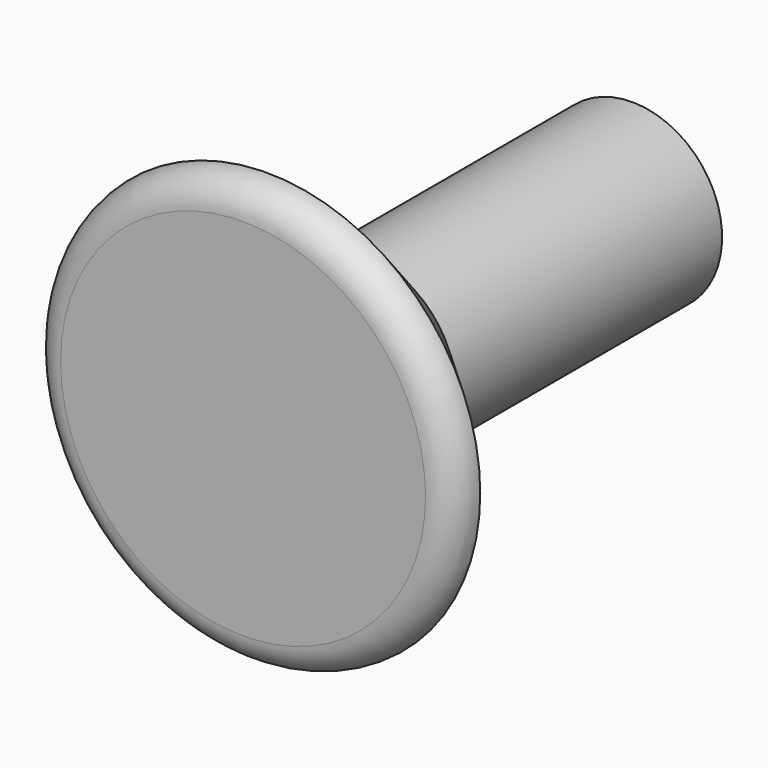
from build123d import *

# Parameters (mm, degrees)
F0_R     = 35
F1_DEPTH = 12.5
F2_R     = 5
F3_SIZE  = 19.99999
F4_R     = 14.7680159512
F5_DEPTH = 55


# Not quite as in the source:
# - a fillet or chamfer is up to 0.001 mm smaller than in the source, because OpenCascade refuses the exact size


with BuildPart() as f1:
    # F0 (on Front) → F1 (new body, symmetric)
    with BuildSketch(Plane.XZ):
        Circle(F0_R)
    extrude(amount=F1_DEPTH, both=True)

    # F2
    f2_edges = [f1.edges().sort_by_distance(p)[0] for p in [
        (-35, -12.5, 0),
    ]]
    fillet(f2_edges, radius=F2_R)

    # F3 (size 20 in the source; OpenCascade refuses exactly that, so slightly less here)
    f3_edges = [f1.edges().sort_by_distance(p)[0] for p in [
        (-35, 12.5, 0),
    ]]
    chamfer(f3_edges, length=F3_SIZE)

    # F4 (on face) → F5 (join)
    with BuildSketch(Plane(origin=(0, 12.5, 0), x_dir=(-1, 0, 0), z_dir=(0, 1, 0))):
        Circle(F4_R)
    extrude(amount=F5_DEPTH)


solid = f1.part
